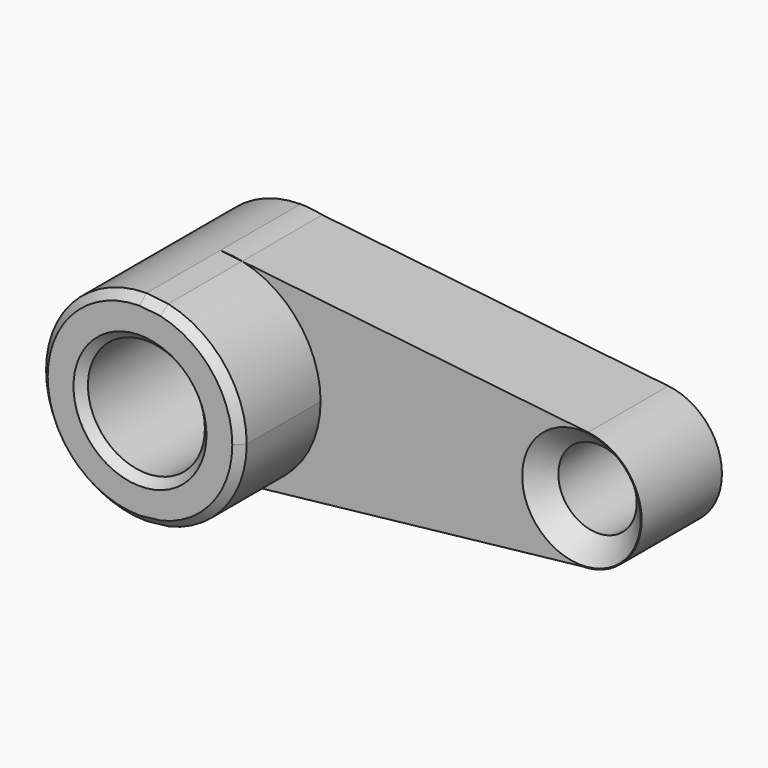
from build123d import *

# Parameters (mm, degrees)
F0_R       = 14.5692591233
F0_R_2     = 9.7754481422
F1_DEPTH   = 25
F2_DEPTH   = 50
F3_C1_SIZE = 2
F3_C2_SIZE = 2
F3_C3_SIZE = 1.9999
F3_C4_SIZE = 1.9999
F3_C5_SIZE = 1.9999
F4_SIZE    = 5


# Not quite as in the source:
# - a fillet or chamfer is up to 0.001 mm smaller than in the source, because OpenCascade refuses the exact size


with BuildPart() as f1:
    # F0 (on Front) → F1 (new body)
    with BuildSketch(Plane.XZ):
        with BuildLine():
            Line((5.4392563459, 24.4011165811), (0, 25))
            ThreePointArc((0, 25), (-25, 0), (0, -25))
            Line((0, -25), (5.487804878, -24.3902439024))
            ThreePointArc((5.487804878, -24.3902439024), (19.5217202361, -15.6173761889), (25, 0))
            ThreePointArc((25, 0), (19.5061709293, 15.6367930113), (5.4392563459, 24.4011165811))
        make_face()
        Circle(F0_R, mode=Mode.SUBTRACT)
        with BuildLine():
            ThreePointArc((5.4392563459, 24.4011165811), (2.7360633648, 24.8498281134), (0, 25))
            Line((0, 25), (5.4392563459, 24.4011165811))
        make_face()
        with BuildLine():
            Line((5.487804878, -24.3902439024), (0, -25))
            ThreePointArc((0, -25), (2.7607881519, -24.8470933668), (5.487804878, -24.3902439024))
        make_face()
        with BuildLine():
            Line((91.6416380189, 14.909896868), (5.4392563459, 24.4011165811))
            ThreePointArc((5.4392563459, 24.4011165811), (19.5061709293, 15.6367930113), (25, 0))
            ThreePointArc((25, 0), (19.5217202361, -15.6173761889), (5.487804878, -24.3902439024))
            Line((5.487804878, -24.3902439024), (90, -15))
            ThreePointArc((90, -15), (75.0225427221, 0.8220544324), (91.6416380189, 14.909896868))
        make_face()
        with BuildLine():
            ThreePointArc((105, 0), (101.1719418698, 10.0093813424), (91.6416380189, 14.909896868))
            ThreePointArc((91.6416380189, 14.909896868), (75.0225427221, 0.8220544324), (90, -15))
            ThreePointArc((90, -15), (100.6066017178, -10.6066017178), (105, 0))
        make_face()
        with Locations((90, 0)):
            Circle(F0_R_2, mode=Mode.SUBTRACT)
    extrude(amount=F1_DEPTH)

    # F0 (on Front) → F2 (join)
    with BuildSketch(Plane.XZ):
        with BuildLine():
            Line((5.4392563459, 24.4011165811), (0, 25))
            ThreePointArc((0, 25), (-25, 0), (0, -25))
            Line((0, -25), (5.487804878, -24.3902439024))
            ThreePointArc((5.487804878, -24.3902439024), (19.5217202361, -15.6173761889), (25, 0))
            ThreePointArc((25, 0), (19.5061709293, 15.6367930113), (5.4392563459, 24.4011165811))
        make_face()
        Circle(F0_R, mode=Mode.SUBTRACT)
    extrude(amount=F2_DEPTH)

    # F3: chamfer of 2 on 5 edges, made by hand

    # F3_c1
    f3_c1_edges = [f1.edges().sort_by_distance(p)[0] for p in [
        (-14.5692591233, -50, 0),
    ]]
    chamfer(f3_c1_edges, length=F3_C1_SIZE)

    # F3_c2
    f3_c2_edges = [f1.edges().sort_by_distance(p)[0] for p in [
        (-25, -50, 0),
    ]]
    chamfer(f3_c2_edges, length=F3_C2_SIZE)

    # F3_c3 (size 2 in the source; OpenCascade refuses exactly that, so slightly less here)
    f3_c3_edges = [f1.edges().sort_by_distance(p)[0] for p in [
        (3.7377861737, -50, -24.5846904251),
    ]]
    chamfer(f3_c3_edges, length=F3_C3_SIZE)

    # F3_c4 (size 2 in the source; OpenCascade refuses exactly that, so slightly less here)
    f3_c4_edges = [f1.edges().sort_by_distance(p)[0] for p in [
        (3.7136212975, -50, 24.591115756),
    ]]
    chamfer(f3_c4_edges, length=F3_C4_SIZE)

    # F3_c5 (size 2 in the source; OpenCascade refuses exactly that, so slightly less here)
    f3_c5_edges = [f1.edges().sort_by_distance(p)[0] for p in [
        (24.9999950028, -50, 0.0158069943),
    ]]
    chamfer(f3_c5_edges, length=F3_C5_SIZE)

    # F4
    f4_edges = [f1.edges().sort_by_distance(p)[0] for p in [
        (80.224552, -25, 0),
    ]]
    chamfer(f4_edges, length=F4_SIZE)


solid = f1.part
